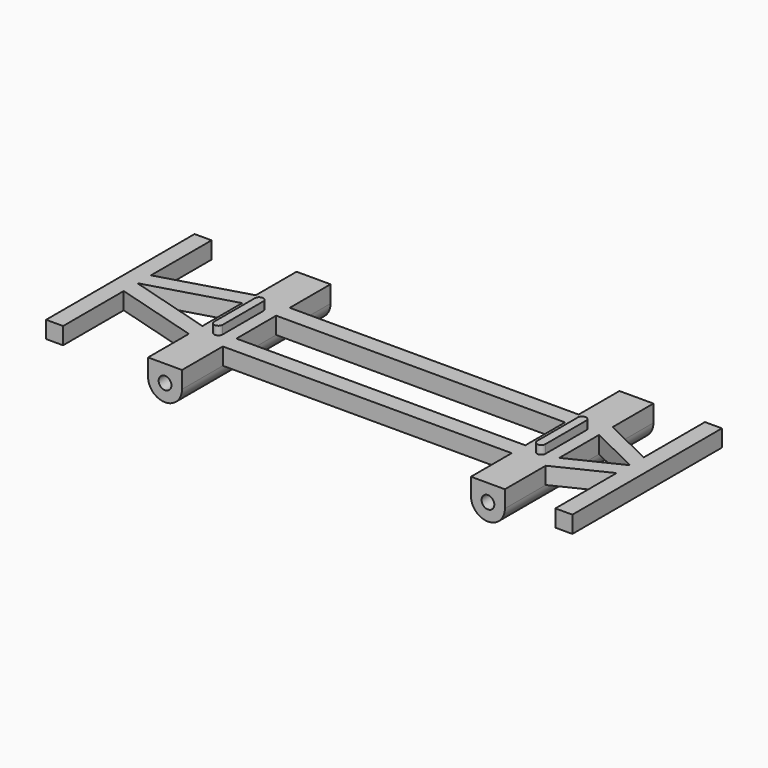
from build123d import *

# Parameters (mm, degrees)
F1_DEPTH  = 2
F3_DEPTH  = 1
F5_DEPTH  = 21.8461783077
F6_W      = 4
F6_H      = 21.8461783077
F7_DEPTH  = 2
F8_R      = 1.99999
F10_R     = 0.75
F9_R      = 0.75
F11_DEPTH = 21.9240891538


# Not quite as in the source:
# - a fillet or chamfer is up to 0.001 mm smaller than in the source, because OpenCascade refuses the exact size


with BuildPart() as f1:
    # F0 (on Top) → F1 (new body)
    with BuildSketch(Plane.XY):
        Polygon((0, -11), (0, 0), (0, 11), (-2, 11), (-2, 2), (-8, 4.9230891538), (-8, 10.9230891538), (-12, 10.9230891538), (-12, 4.9230891538), (-29, 4.9230891538), (-46, 4.9230891538), (-46, 10.9230891538), (-50, 10.9230891538), (-50, 4.9230891538), (-60, 2), (-60, 10.9230891538), (-62, 10.9230891538), (-62, -10.9230891538), (-60, -10.9230891538), (-60, -2), (-50, -4.9230891538), (-50, -10.9230891538), (-46, -10.9230891538), (-46, -4.9230891538), (-29, -4.9230891538), (-12, -4.9230891538), (-12, -10.9230891538), (-8, -10.9230891538), (-8, -4.9230891538), (-2, -2), (-2, -11), align=None)
        Polygon((-60, 0), (-50, 2.9230891538), (-50, -2.9230891538), align=None, mode=Mode.SUBTRACT)
        Polygon((-12, 2.9230891538), (-12, 0), (-12, -2.9230891538), (-29, -2.9230891538), (-46, -2.9230891538), (-46, 0), (-46, 2.9230891538), (-29, 2.9230891538), align=None, mode=Mode.SUBTRACT)
        Polygon((-8, 2.9230891538), (-2, 0), (-8, -2.9230891538), (-8, 0), align=None, mode=Mode.SUBTRACT)
    extrude(amount=F1_DEPTH)

    # F2 (on face) → F3 (join)
    with BuildSketch(Plane.XY.offset(2)):
        with BuildLine():
            Line((-47.5, -3.0769108462), (-47.5, 2.9230891538))
            ThreePointArc((-47.5, 2.9230891538), (-48, 3.4230891538), (-48.5, 2.9230891538))
            Line((-48.5, 2.9230891538), (-48.5, -3.0769108462))
            ThreePointArc((-48.5, -3.0769108462), (-48, -3.5769108462), (-47.5, -3.0769108462))
        make_face()
        with BuildLine():
            Line((-9.5, -3.0769108462), (-9.5, 2.9230891538))
            ThreePointArc((-9.5, 2.9230891538), (-10, 3.4230891538), (-10.5, 2.9230891538))
            Line((-10.5, 2.9230891538), (-10.5, -3.0769108462))
            ThreePointArc((-10.5, -3.0769108462), (-10, -3.5769108462), (-9.5, -3.0769108462))
        make_face()
    extrude(amount=F3_DEPTH)

    # F4 (on face) → F5 (join, through all)
    with BuildSketch(Plane.XZ.offset(10.9230891538)):
        with BuildLine():
            Line((-46, 0), (-50, 0))
            ThreePointArc((-50, 0), (-48, -2), (-46, 0))
        make_face()
    extrude(amount=-F5_DEPTH)

    # F6 (on face) → F7 (join)
    with BuildSketch(Plane(origin=(0, 0, 0), x_dir=(1, 0, 0), z_dir=(0, 0, -1))):
        with Locations((-10, 0)):
            Rectangle(F6_W, F6_H)
    extrude(amount=F7_DEPTH)

    # F8 (radius 2 in the source; OpenCascade refuses exactly that, so slightly less here)
    f8_edges = [f1.edges().sort_by_distance(p)[0] for p in [
        (-12, 0, -2),
        (-8, 0, -2),
    ]]
    fillet(f8_edges, radius=F8_R)

    # F10 (on face) + F9 (on face) → F11 (cut, through all)
    with BuildSketch(Plane.XZ.offset(10.9230891538)):
        with Locations((-10, 0)):
            Circle(F10_R)
    with BuildSketch(Plane.XZ.offset(10.9230891538)):
        with Locations((-48, 0)):
            Circle(F9_R)
    extrude(amount=-F11_DEPTH, mode=Mode.SUBTRACT)


solid = f1.part
